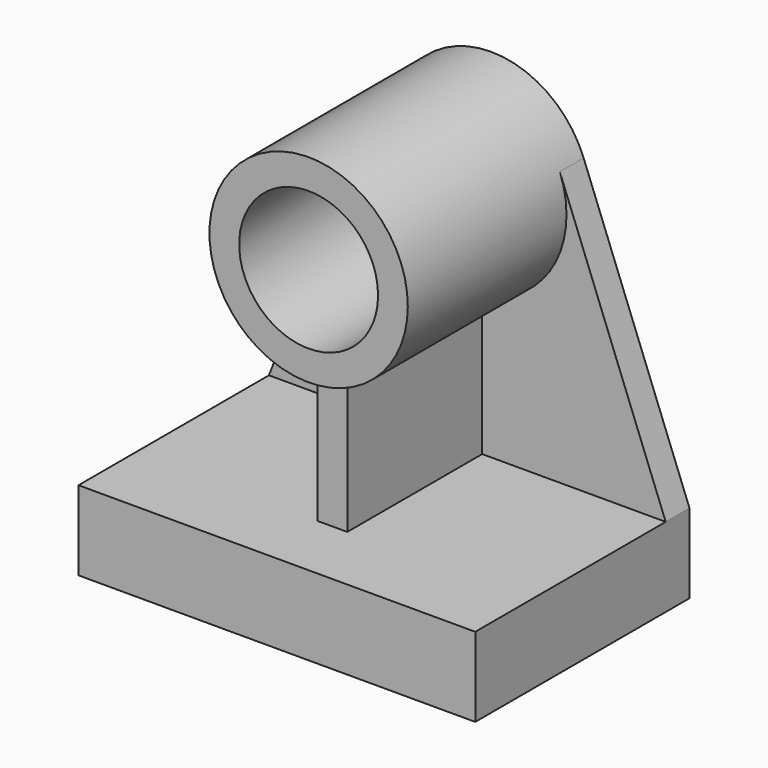
from build123d import *

# Parameters (mm, degrees)
F2_DEPTH  = 19.05
F3_W      = 254
F3_H      = 50.8
F4_DEPTH  = 152.4
F5_W      = 19.05
F5_H      = 152.4
F6_DEPTH  = 107.95
F7_R      = 63.5
F8_DEPTH  = 127
F9_R      = 44.45
F10_DEPTH = 146.051


# Not quite as in the source:
# - a variable given as a bare number and used for a length is read in inches; the dataset says mm whatever the document's units were


with BuildPart() as f2:
    # F1 (on Front) → F2 (new body)
    with BuildSketch(Plane.XZ):
        with BuildLine():
            Line((-254, 0), (0, 0))
            Line((0, 0), (0, 50.8))
            Line((0, 50.8), (-67.7722531834, 226.0981223472))
            ThreePointArc((-67.7722531834, 226.0981223472), (-127, 266.7), (-186.2277468166, 226.0981223472))
            Line((-186.2277468166, 226.0981223472), (-254, 50.8))
            Line((-254, 50.8), (-254, 0))
        make_face()
    extrude(amount=F2_DEPTH)

    # F3 (on face) → F4 (join)
    with BuildSketch(Plane.XZ.offset(19.05)):
        with Locations((-127, 25.4)):
            Rectangle(F3_W, F3_H)
    extrude(amount=F4_DEPTH)

    # F5 (on face) → F6 (join)
    with BuildSketch(Plane.XZ.offset(19.05)):
        with Locations((-127, 127)):
            Rectangle(F5_W, F5_H)
    extrude(amount=F6_DEPTH)

    # F7 (on face) → F8 (join)
    with BuildSketch(Plane.XZ.offset(19.05)):
        with Locations((-127, 203.2)):
            Circle(F7_R)
    extrude(amount=F8_DEPTH)

    # F9 (on face) → F10 (cut, through all)
    with BuildSketch(Plane.XZ.offset(146.05)):
        with Locations((-127, 203.2)):
            Circle(F9_R)
    extrude(amount=-F10_DEPTH, mode=Mode.SUBTRACT)


solid = f2.part
